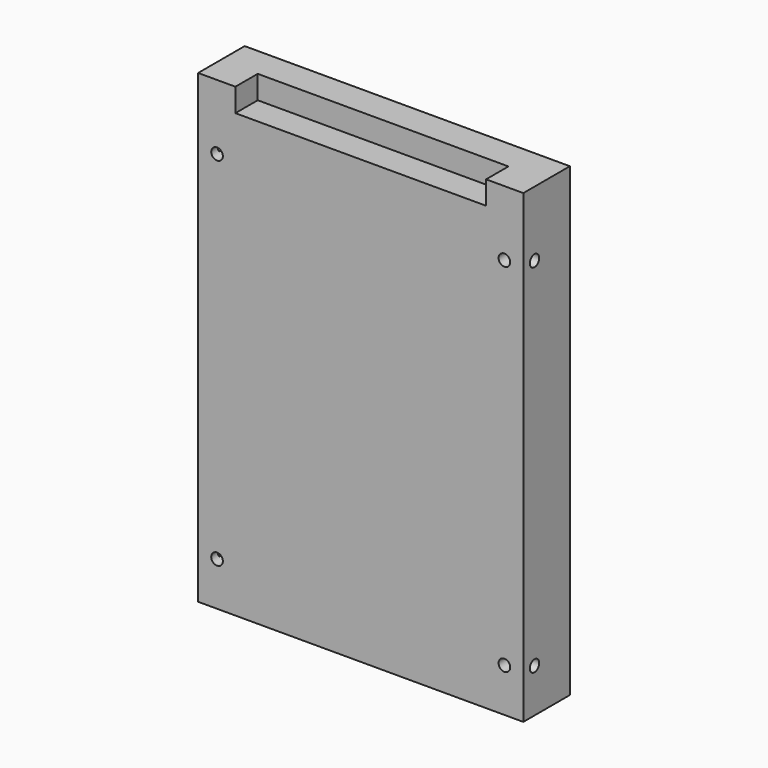
from build123d import *

# Parameters (mm, degrees)
F0_W     = 69.85
F0_H     = 100
F1_DEPTH = 12.5
F2_R     = 1.25
F2_W     = 53.85
F2_H     = 5
F3_DEPTH = 6
F4_R     = 1.25
F5_DEPTH = 3


# Not quite as in the source:
# - a pattern or mirror of a feature is missing from the dataset's text; its kind, count and spacing are read off the source's solid


with BuildPart() as f1:
    # F0 (on Front) → F1 (new body)
    with BuildSketch(Plane.XZ):
        with Locations((34.925, 50)):
            Rectangle(F0_W, F0_H)
    extrude(amount=F1_DEPTH)

    # F2 (on face) → F3 (cut)
    with BuildSketch(Plane.XZ.offset(12.5)):
        with Locations((4.065, 9.4)):
            Circle(F2_R)
        with Locations((4.065, 86)):
            Circle(F2_R)
        with Locations((65.785, 9.4)):
            Circle(F2_R)
        with Locations((65.785, 86)):
            Circle(F2_R)
        with Locations((34.925, 97.5)):
            Rectangle(F2_W, F2_H)
    extrude(amount=-F3_DEPTH, mode=Mode.SUBTRACT)

    # F4 (on face) → F5 (cut)
    with BuildSketch(Plane(origin=(0, 0, 0), x_dir=(0, -1, 0), z_dir=(-1, 0, 0))):
        with Locations((9.5, 86)):
            Circle(F4_R)
        with Locations((9.5, 9.4)):
            Circle(F4_R)
    f5 = extrude(amount=-F5_DEPTH, mode=Mode.SUBTRACT)

    # F5_copies: F5 across plane
    add(f5.mirror(Plane(origin=(34.925, 0, 0), x_dir=(0, 0, 1), z_dir=(1, 0, 0))), mode=Mode.SUBTRACT)


solid = f1.part
